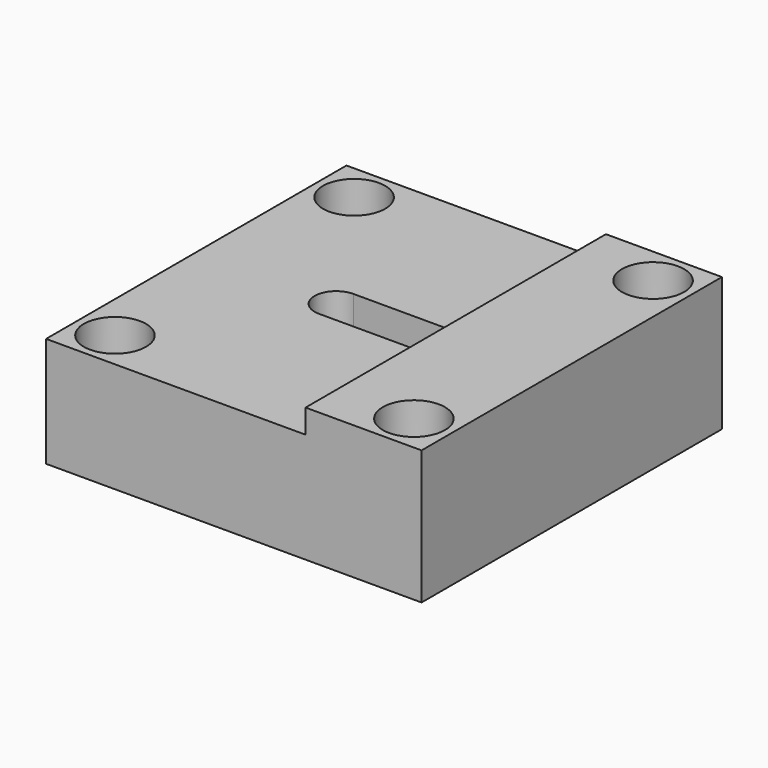
from build123d import *

# Parameters (mm, degrees)
F0_W     = 12.319
F0_H     = 39.878
F0_R     = 3.302
F0_W_2   = 27.559
F1_DEPTH = 11.684
F0_R_2   = 2.159
F2_DEPTH = 5.842
F3_DEPTH = 14.224
F5_DEPTH = 25.4
F6_DEPTH = 5.842


# Not quite as in the source:
# - a feature names something its author has since deleted; it is built from what else it names


with BuildPart() as f1:
    # F0 (on Top) → F1 (new body)
    with BuildSketch(Plane.XY):
        with Locations((13.7795, 0)):
            Rectangle(F0_W, F0_H)
        with Locations((15.875, -15.875)):
            Circle(F0_R, mode=Mode.SUBTRACT)
        with Locations((15.875, 15.875)):
            Circle(F0_R, mode=Mode.SUBTRACT)
        with Locations((-6.1595, 0)):
            Rectangle(F0_W_2, F0_H)
        with Locations((-15.875, -15.875)):
            Circle(F0_R, mode=Mode.SUBTRACT)
        with Locations((-15.875, 15.875)):
            Circle(F0_R, mode=Mode.SUBTRACT)
    extrude(amount=F1_DEPTH)

    # F0 (on Top) → F2 (join)
    with BuildSketch(Plane.XY):
        with Locations((-15.875, 15.875)):
            Circle(F0_R)
        with Locations((-15.875, 15.875)):
            Circle(F0_R_2, mode=Mode.SUBTRACT)
        with Locations((15.875, 15.875)):
            Circle(F0_R)
        with Locations((15.875, 15.875)):
            Circle(F0_R_2, mode=Mode.SUBTRACT)
        with Locations((15.875, -15.875)):
            Circle(F0_R)
        with Locations((15.875, -15.875)):
            Circle(F0_R_2, mode=Mode.SUBTRACT)
        with Locations((-15.875, -15.875)):
            Circle(F0_R)
        with Locations((-15.875, -15.875)):
            Circle(F0_R_2, mode=Mode.SUBTRACT)
    extrude(amount=F2_DEPTH)

    # F0 (on Top) → F3 (join)
    with BuildSketch(Plane.XY):
        with Locations((13.7795, 0)):
            Rectangle(F0_W, F0_H)
        with Locations((15.875, -15.875)):
            Circle(F0_R, mode=Mode.SUBTRACT)
        with Locations((15.875, 15.875)):
            Circle(F0_R, mode=Mode.SUBTRACT)
    extrude(amount=F3_DEPTH)

    # F4 (on face) → F5 (cut)
    with BuildSketch(Plane(origin=(0, 0, 0), x_dir=(1, 0, 0), z_dir=(0, 0, -1))):
        with BuildLine():
            ThreePointArc((-2.794, 0), (-3.4635538982, 1.6164461018), (-5.08, 2.286))
            ThreePointArc((-5.08, 2.286), (-7.366, 0), (-5.08, -2.286))
            ThreePointArc((-5.08, -2.286), (-3.4635538982, -1.6164461018), (-2.794, 0))
        make_face()
        with BuildLine():
            ThreePointArc((7.366, 0), (6.6964461018, 1.6164461018), (5.08, 2.286))
            ThreePointArc((5.08, 2.286), (2.794, 0), (5.08, -2.286))
            ThreePointArc((5.08, -2.286), (6.6964461018, -1.6164461018), (7.366, 0))
        make_face()
        with BuildLine():
            ThreePointArc((-1.27, 0), (-1.4655166344, 1.2048277885), (-2.032, 2.286))
            Line((-2.032, 2.286), (-5.08, 2.286))
            ThreePointArc((-5.08, 2.286), (-3.4635538982, 1.6164461018), (-2.794, 0))
            ThreePointArc((-2.794, 0), (-3.4635538982, -1.6164461018), (-5.08, -2.286))
            Line((-5.08, -2.286), (-2.032, -2.286))
            ThreePointArc((-2.032, -2.286), (-1.4655166344, -1.2048277885), (-1.27, 0))
        make_face()
        with BuildLine():
            ThreePointArc((2.032, -2.286), (1.27, 0), (2.032, 2.286))
            Line((2.032, 2.286), (-2.032, 2.286))
            ThreePointArc((-2.032, 2.286), (-1.4655166344, 1.2048277885), (-1.27, 0))
            ThreePointArc((-1.27, 0), (-1.4655166344, -1.2048277885), (-2.032, -2.286))
            Line((-2.032, -2.286), (2.032, -2.286))
        make_face()
        with BuildLine():
            Line((5.08, 2.286), (2.032, 2.286))
            ThreePointArc((2.032, 2.286), (1.27, 0), (2.032, -2.286))
            Line((2.032, -2.286), (5.08, -2.286))
            ThreePointArc((5.08, -2.286), (2.794, 0), (5.08, 2.286))
        make_face()
    extrude(amount=-F5_DEPTH, mode=Mode.SUBTRACT)

    # F4 (on face) → F6 (cut)
    with BuildSketch(Plane(origin=(0, 0, 0), x_dir=(1, 0, 0), z_dir=(0, 0, -1))):
        with BuildLine():
            ThreePointArc((-1.27, 0), (-1.4655166344, 1.2048277885), (-2.032, 2.286))
            Line((-2.032, 2.286), (-5.08, 2.286))
            ThreePointArc((-5.08, 2.286), (-3.4635538982, 1.6164461018), (-2.794, 0))
            ThreePointArc((-2.794, 0), (-3.4635538982, -1.6164461018), (-5.08, -2.286))
            Line((-5.08, -2.286), (-2.032, -2.286))
            ThreePointArc((-2.032, -2.286), (-1.4655166344, -1.2048277885), (-1.27, 0))
        make_face()
        with BuildLine():
            ThreePointArc((-2.032, 2.286), (-3.3761162011, 3.4077675977), (-5.08, 3.81))
            ThreePointArc((-5.08, 3.81), (-8.89, 0), (-5.08, -3.81))
            ThreePointArc((-5.08, -3.81), (-3.3761162011, -3.4077675977), (-2.032, -2.286))
            Line((-2.032, -2.286), (-5.08, -2.286))
            ThreePointArc((-5.08, -2.286), (-7.366, 0), (-5.08, 2.286))
            Line((-5.08, 2.286), (-2.032, 2.286))
        make_face()
        with BuildLine():
            ThreePointArc((2.032, 2.286), (3.3761162011, 3.4077675977), (5.08, 3.81))
            Line((5.08, 3.81), (-5.08, 3.81))
            ThreePointArc((-5.08, 3.81), (-3.3761162011, 3.4077675977), (-2.032, 2.286))
            Line((-2.032, 2.286), (2.032, 2.286))
        make_face()
        with BuildLine():
            ThreePointArc((2.032, -2.286), (1.27, 0), (2.032, 2.286))
            Line((2.032, 2.286), (-2.032, 2.286))
            ThreePointArc((-2.032, 2.286), (-1.4655166344, 1.2048277885), (-1.27, 0))
            ThreePointArc((-1.27, 0), (-1.4655166344, -1.2048277885), (-2.032, -2.286))
            Line((-2.032, -2.286), (2.032, -2.286))
        make_face()
        with BuildLine():
            Line((5.08, 2.286), (2.032, 2.286))
            ThreePointArc((2.032, 2.286), (1.27, 0), (2.032, -2.286))
            Line((2.032, -2.286), (5.08, -2.286))
            ThreePointArc((5.08, -2.286), (2.794, 0), (5.08, 2.286))
        make_face()
        with BuildLine():
            ThreePointArc((5.08, -3.81), (7.7740768363, -2.6940768363), (8.89, 0))
            ThreePointArc((8.89, 0), (7.7740768363, 2.6940768363), (5.08, 3.81))
            ThreePointArc((5.08, 3.81), (3.3761162011, 3.4077675977), (2.032, 2.286))
            Line((2.032, 2.286), (5.08, 2.286))
            ThreePointArc((5.08, 2.286), (6.6964461018, 1.6164461018), (7.366, 0))
            ThreePointArc((7.366, 0), (6.6964461018, -1.6164461018), (5.08, -2.286))
            Line((5.08, -2.286), (2.032, -2.286))
            ThreePointArc((2.032, -2.286), (3.3761162011, -3.4077675977), (5.08, -3.81))
        make_face()
        with BuildLine():
            Line((-5.08, -3.81), (5.08, -3.81))
            ThreePointArc((5.08, -3.81), (3.3761162011, -3.4077675977), (2.032, -2.286))
            Line((2.032, -2.286), (-2.032, -2.286))
            ThreePointArc((-2.032, -2.286), (-3.3761162011, -3.4077675977), (-5.08, -3.81))
        make_face()
    extrude(amount=-F6_DEPTH, mode=Mode.SUBTRACT)


solid = f1.part
